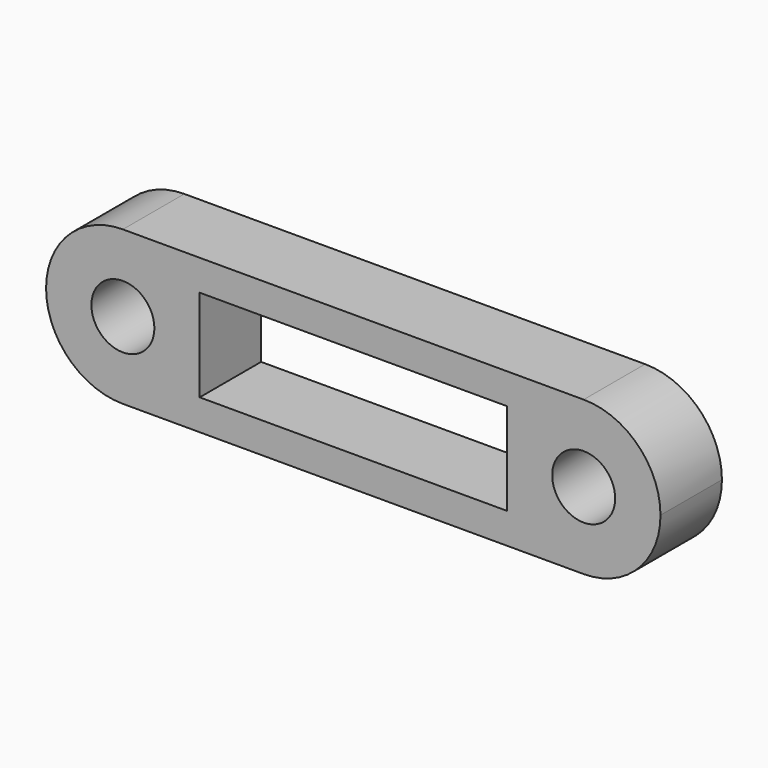
from build123d import *

# Parameters (mm, degrees)
F0_W     = 40
F0_H     = 5
F1_DEPTH = 10
F2_R     = 2.05
F3_DEPTH = 25
F4_R     = 2.05
F5_DEPTH = 25
F6_R     = 4.99999
F7_W     = 20
F7_H     = 6
F8_DEPTH = 25


# Not quite as in the source:
# - a fillet or chamfer is up to 0.001 mm smaller than in the source, because OpenCascade refuses the exact size


with BuildPart() as f1:
    # F0 (on Top) → F1 (new body)
    with BuildSketch(Plane.XY):
        with Locations((20, 2.5)):
            Rectangle(F0_W, F0_H)
    extrude(amount=F1_DEPTH)

    # F2 (on face) → F3 (cut)
    with BuildSketch(Plane.XZ):
        with Locations((5, 5)):
            Circle(F2_R)
    extrude(amount=-F3_DEPTH, mode=Mode.SUBTRACT)

    # F4 (on face) → F5 (cut)
    with BuildSketch(Plane.XZ):
        with Locations((35, 5)):
            Circle(F4_R)
    extrude(amount=-F5_DEPTH, mode=Mode.SUBTRACT)

    # F6 (radius 5 in the source; OpenCascade refuses exactly that, so slightly less here)
    f6_edges = [f1.edges().sort_by_distance(p)[0] for p in [
        (0, 2.5, 10),
        (0, 2.5, 0),
        (40, 2.5, 10),
        (40, 2.5, 0),
    ]]
    fillet(f6_edges, radius=F6_R)

    # F7 (on face) → F8 (cut)
    with BuildSketch(Plane(origin=(0, 5, 0), x_dir=(-1, 0, 0), z_dir=(0, 1, 0))):
        with Locations((-20, 5)):
            Rectangle(F7_W, F7_H)
    extrude(amount=-F8_DEPTH, mode=Mode.SUBTRACT)


solid = f1.part
